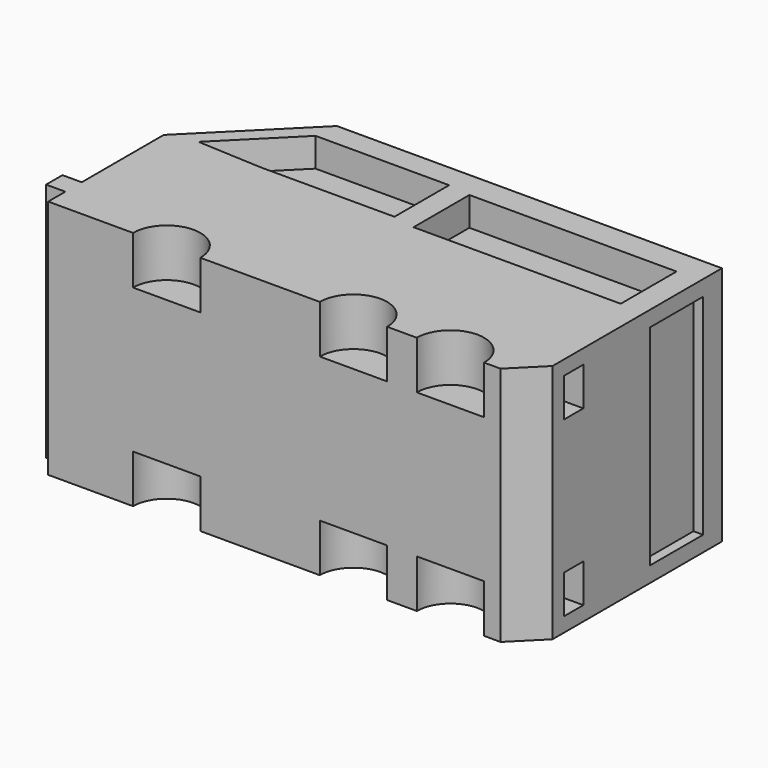
from build123d import *

# Parameters (mm, degrees)
F0_W      = 50
F0_H      = 25
F1_DEPTH  = 12.5
F2_R      = 3.5
F3_DEPTH  = 5
F4_SIZE   = 10
F5_SIZE   = 3
F6_W      = 2.1288916469
F6_H      = 25
F7_DEPTH  = 2
F8_W      = 9.6029471606
F8_H      = 18.9187433571
F9_DEPTH  = 1
F10_W     = 13.8777932152
F10_H     = 7.1009902749
F10_W_2   = 21.5250877663
F10_H_2   = 7.2504867127
F11_DEPTH = 3
F12_W     = 6.9172445219
F12_H     = 21.7759581094
F13_DEPTH = 1
F14_W     = 2.5
F14_H     = 4
F15_DEPTH = 2
F16_W     = 2.5
F16_H     = 5
F17_DEPTH = 2


# Not quite as in the source:
# - a pattern or mirror of a feature is missing from the dataset's text; its kind, count and spacing are read off the source's solid


with BuildPart() as f1:
    # F0 (on Top) → F1 (new body, symmetric)
    with BuildSketch(Plane.XY):
        with Locations((1.3995850459, -7.8662077549)):
            Rectangle(F0_W, F0_H)
    extrude(amount=F1_DEPTH, both=True)

    # F2 (on face) → F3 (cut)
    with BuildSketch(Plane.XY.offset(12.5)):
        with Locations((-11.2899886444, -20.3662077549)):
            Circle(F2_R)
        with Locations((8.1175947562, -20.3662077549)):
            Circle(F2_R)
        with Locations((18.194610253, -20.3662077549)):
            Circle(F2_R)
    f3 = extrude(amount=-F3_DEPTH, mode=Mode.SUBTRACT)

    # F3_copies: F3 across plane
    add(f3.mirror(Plane(origin=(0, 0, 0), x_dir=(-1, 0, 0), z_dir=(0, 0, -1))), mode=Mode.SUBTRACT)

    # F4
    f4_edges = [f1.edges().sort_by_distance(p)[0] for p in [
        (-23.600415, 4.633792, 0),
    ]]
    chamfer(f4_edges, length=F4_SIZE)

    # F5
    f5_edges = [f1.edges().sort_by_distance(p)[0] for p in [
        (26.399585, -20.366208, 0),
    ]]
    chamfer(f5_edges, length=F5_SIZE)

    # F6 (on face) → F7 (join)
    with BuildSketch(Plane(origin=(-23.6004149541, 0, 0), x_dir=(0, -1, 0), z_dir=(-1, 0, 0))):
        with Locations((17.0801598579, 0)):
            Rectangle(F6_W, F6_H)
    extrude(amount=F7_DEPTH)

    # F8 (on face) → F9 (cut, symmetric)
    with BuildSketch(Plane(origin=(-9.1171035996, 9.1171035996, 0), x_dir=(-0.7071067812, -0.7071067812, 0), z_dir=(-0.7071067812, 0.7071067812, 0))):
        with Locations((13.4759480134, -0.2812528983)):
            Rectangle(F8_W, F8_H)
    extrude(amount=F9_DEPTH, both=True, mode=Mode.SUBTRACT)

    # F10 (on face) → F11 (cut)
    with BuildSketch(Plane.XY.offset(12.5)):
        with Locations((-6.9388966076, -1.3492055004)):
            Rectangle(F10_W, F10_H)
        Polygon((-13.8777932152, -4.8997006379), (-13.8777932152, 2.201289637), (-20.6305080792, -4.551425227), align=None)
        with Locations((13.1223001517, -1.7409643986)):
            Rectangle(F10_W_2, F10_H_2)
    f11 = extrude(amount=-F11_DEPTH, mode=Mode.SUBTRACT)

    # F11_copies: F11 across plane
    add(f11.mirror(Plane(origin=(0, 0, 0), x_dir=(-1, 0, 0), z_dir=(0, 0, -1))), mode=Mode.SUBTRACT)

    # F12 (on face) → F13 (cut, symmetric)
    with BuildSketch(Plane.YZ.offset(26.3995850459)):
        with Locations((-1.2673075544, -2.09453e-05)):
            Rectangle(F12_W, F12_H)
    extrude(amount=F13_DEPTH, both=True, mode=Mode.SUBTRACT)

    # F14 (on face) → F15 (cut)
    with BuildSketch(Plane.YZ.offset(26.3995850459)):
        with Locations((-14.6162077549, -9)):
            Rectangle(F14_W, F14_H)
        with Locations((-14.6162077549, 9)):
            Rectangle(F14_W, F14_H)
    extrude(amount=-F15_DEPTH, mode=Mode.SUBTRACT)

    # F16 (on face) → F17 (cut)
    with BuildSketch(Plane(origin=(-23.6004149541, 0, 0), x_dir=(0, -1, 0), z_dir=(-1, 0, 0))):
        with Locations((13.2657140344, 8.25)):
            Rectangle(F16_W, F16_H)
        with Locations((13.2657140344, -8.25)):
            Rectangle(F16_W, F16_H)
    extrude(amount=-F17_DEPTH, mode=Mode.SUBTRACT)


solid = f1.part
